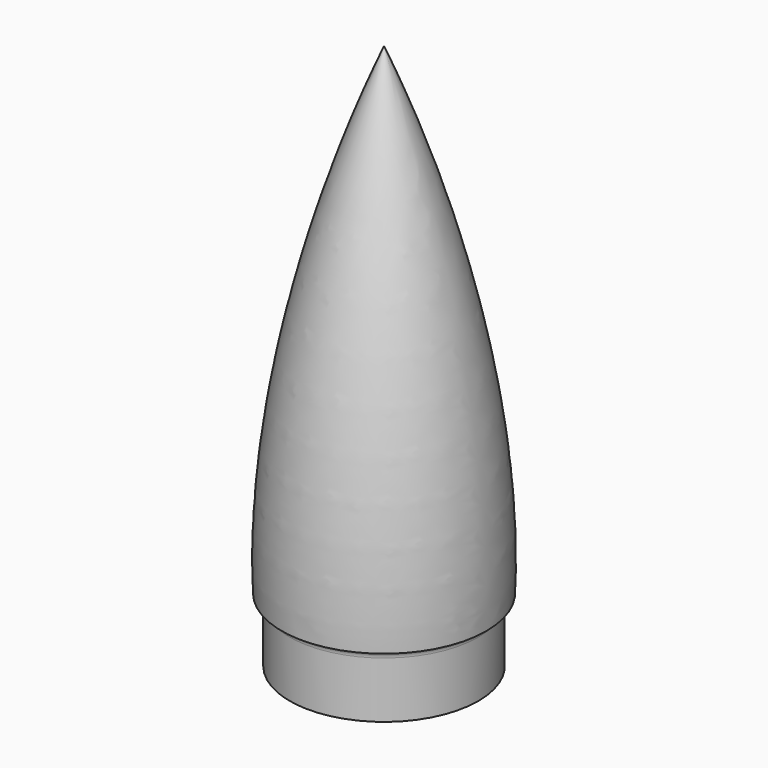
from build123d import *

# Parameters (mm, degrees)
F2_R = 0.99999


# Not quite as in the source:
# - a fillet or chamfer is up to 0.001 mm smaller than in the source, because OpenCascade refuses the exact size


with BuildPart() as f1:
    # F0 (on Front) → F1 (revolve)
    with BuildSketch(Plane.XZ):
        with BuildLine():
            add(Edge.make_bspline(
                [(0, 68), (7.9392548651, 49.6992245317), (13.5644692928, 26.8943756819), (12.75, 8)],
                knots=[0, 0, 0, 0, 61.3397301918, 61.3397301918, 61.3397301918, 61.3397301918], degree=3))
            Line((0, 68), (0, 65.4882118106))
            add(Edge.make_bspline(
                [(0, 65.4882118106), (6.5256207423, 48.9649383531), (11.3890371188, 30.6826956818), (11.7690293485, 13.1080830189)],
                knots=[0, 0, 0, 0, 53.4733274618, 53.4733274618, 53.4733274618, 53.4733274618], degree=3))
            add(Edge.make_bspline(
                [(11.7690293485, 13.1080830189), (11.8060056748, 11.3979306507), (11.8005290471, 9.6944787382), (11.75, 8)],
                knots=[53.4733274618, 53.4733274618, 53.4733274618, 53.4733274618, 58.6767159713, 58.6767159713, 58.6767159713, 58.6767159713], degree=3))
            Line((11.75, 8), (12.75, 8))
        make_face()
        Polygon((11.75, 0), (11.75, 8), (6.7701976789, 8), (6.6109633365, 8), (0, 8), (0, 7), (0.5, 7), (0.5, 0), align=None)
        with BuildLine():
            Line((6.7701976789, 8), (11.75, 8))
            add(Edge.make_bspline(
                [(11.7690293485, 13.1080830189), (11.8060056748, 11.3979306507), (11.8005290471, 9.6944787382), (11.75, 8)],
                knots=[53.4733274618, 53.4733274618, 53.4733274618, 53.4733274618, 58.6767159713, 58.6767159713, 58.6767159713, 58.6767159713], degree=3))
            ThreePointArc((11.7690293485, 13.1080830189), (10.3437403955, 9.5028879839), (6.7701976789, 8))
        make_face()
    revolve(axis=Axis((0, 0, 36.7441059053), (0, 0, 1)))

    # F2 (radius 1 in the source; OpenCascade refuses exactly that, so slightly less here)
    f2_edges = [f1.edges().sort_by_distance(p)[0] for p in [
        (-11.75, 0, 8),
    ]]
    fillet(f2_edges, radius=F2_R)


solid = f1.part
